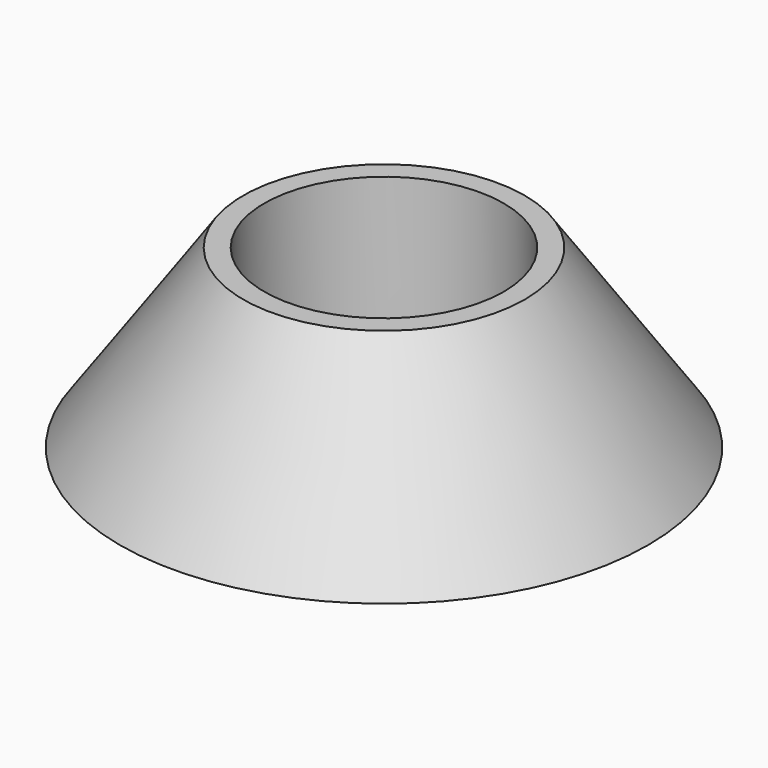
from build123d import *

# Parameters (mm, degrees)
F0_R     = 37.5
F1_DEPTH = 25
F1_TAPER = 35
F2_R     = 17
F3_DEPTH = 20


with BuildPart() as f1:
    # F0 (on Top) → F1 (new body)
    with BuildSketch(Plane.XY):
        Circle(F0_R)
    extrude(amount=F1_DEPTH, taper=F1_TAPER)

    # F2 (on face) → F3 (cut)
    with BuildSketch(Plane.XY.offset(25)):
        Circle(F2_R)
    extrude(amount=-F3_DEPTH, mode=Mode.SUBTRACT)


solid = f1.part
